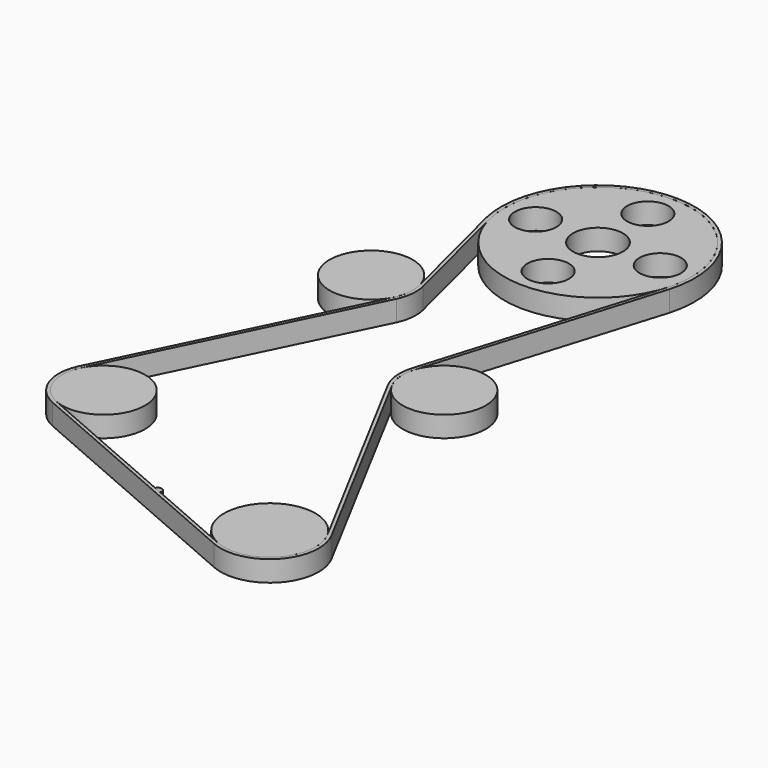
from build123d import *

# Parameters (mm, degrees)
F0_R     = 10
F1_DEPTH = 5
F0_R_2   = 11
F0_R_3   = 22.5
F0_R_4   = 5
F0_R_5   = 6
F3_DEPTH = 5
F4_W     = 2
F4_H     = 5
F5_DEPTH = 1
F6_R     = 0.99999


# Not quite as in the source:
# - a fillet or chamfer is up to 0.001 mm smaller than in the source, because OpenCascade refuses the exact size


with BuildPart() as f1:
    # F0 (on Top) → F1 (new body)
    with BuildSketch(Plane.XY):
        with Locations((-25, 43)):
            Circle(F0_R)
    extrude(amount=F1_DEPTH)


with BuildPart() as f1b:
    # F0 (on Top) → F1, piece 2 (new body)
    with BuildSketch(Plane.XY):
        with Locations((15, 15)):
            Circle(F0_R)
    extrude(amount=F1_DEPTH)


with BuildPart() as f1c:
    # F0 (on Top) → F1, piece 3 (new body)
    with BuildSketch(Plane.XY):
        with Locations((-35, -25)):
            Circle(F0_R)
    extrude(amount=F1_DEPTH)


with BuildPart() as f1d:
    # F0 (on Top) → F1, piece 4 (new body)
    with BuildSketch(Plane.XY):
        with Locations((25, -50)):
            Circle(F0_R_2)
    extrude(amount=F1_DEPTH)


with BuildPart() as f1e:
    # F0 (on Top) → F1, piece 5 (new body)
    with BuildSketch(Plane.XY):
        with Locations((0, 80)):
            Circle(F0_R_3)
        with Locations((-15, 80)):
            Circle(F0_R_4, mode=Mode.SUBTRACT)
        with Locations((0, 65)):
            Circle(F0_R_4, mode=Mode.SUBTRACT)
        with Locations((0, 80)):
            Circle(F0_R_5, mode=Mode.SUBTRACT)
        with Locations((15, 80)):
            Circle(F0_R_4, mode=Mode.SUBTRACT)
        with Locations((0, 95)):
            Circle(F0_R_4, mode=Mode.SUBTRACT)
    extrude(amount=F1_DEPTH)


with BuildPart() as f3:
    # F2 (on Top) → F3 (new body)
    with BuildSketch(Plane.XY):
        with BuildLine():
            ThreePointArc((-15.2430288474, 45.1912357077), (-15.0606342981, 41.9004503453), (-15.9579069335, 38.7291039608))
            Line((-15.9579069335, 38.7291039608), (-44.7654605118, -20.3874322777))
            ThreePointArc((-44.7654605118, -20.3874322777), (-45.1089247172, -28.8012683491), (-39.3067273264, -34.9041455833))
            Line((-39.3067273264, -34.9041455833), (20.2945016249, -60.8211961003))
            ThreePointArc((20.2945016249, -60.8211961003), (33.6205994102, -58.0576215975), (35.4792552674, -44.5754991896))
            Line((35.4792552674, -44.5754991896), (6.1192751972, 10.4029654149))
            ThreePointArc((6.1192751972, 10.4029654149), (5.0477785416, 14.0236352918), (5.3952054736, 17.7835089554))
            Line((5.3952054736, 17.7835089554), (22.3791712466, 73.5144241338))
            ThreePointArc((22.3791712466, 73.5144241338), (0.7124099554, 103.2891062958), (-22.7337427856, 74.8944208011))
            Line((-22.7337427856, 74.8944208011), (-15.2430288474, 45.1912357077))
        make_face()
        with BuildLine():
            ThreePointArc((-21.9531850934, 75.0697196577), (0.6879495277, 102.4894803285), (21.6107876845, 73.7371048503))
            Line((21.6107876845, 73.7371048503), (4.6268219115, 18.0061896719))
            ThreePointArc((4.6268219115, 18.0061896719), (4.251600825, 13.9455261151), (5.4088172129, 10.0352026481))
            Line((5.4088172129, 10.0352026481), (34.7687972831, -44.9432619564))
            ThreePointArc((34.7687972831, -44.9432619564), (33.0361519926, -57.5113421672), (20.6135184639, -60.0875556867))
            Line((20.6135184639, -60.0875556867), (-38.9877104874, -34.1705051698))
            ThreePointArc((-38.9877104874, -34.1705051698), (-44.3601154789, -28.5196929159), (-44.0420930665, -20.7291039608))
            Line((-44.0420930665, -20.7291039608), (-15.2345394882, 38.3874322777))
            ThreePointArc((-15.2345394882, 38.3874322777), (-14.2654850419, 41.8124863729), (-14.4624711552, 45.3665345643))
            Line((-14.4624711552, 45.3665345643), (-21.9531850934, 75.0697196577))
        make_face(mode=Mode.SUBTRACT)
    extrude(amount=F3_DEPTH)


with BuildPart() as f5:
    # F4 (on face) → F5 (new body)
    with BuildSketch(Plane(origin=(-18.6956826234, -42.994308311, 0), x_dir=(-0.917050517, 0.3987710487, 0), z_dir=(0.3987710487, 0.917050517, 0))):
        with Locations((-18.5813830942, 2.5)):
            Rectangle(F4_W, F4_H)
    extrude(amount=F5_DEPTH)

    # F6 (radius 1 in the source; OpenCascade refuses exactly that, so slightly less here)
    f6_edges = [f5.edges().sort_by_distance(p)[0] for p in [
        (-2.173895, -49.088204, 2.5),
        (-0.339794, -49.885746, 2.5),
    ]]
    fillet(f6_edges, radius=F6_R)


solid = Compound([f1.part, f1b.part, f1c.part, f1d.part, f1e.part, f3.part, f5.part])
